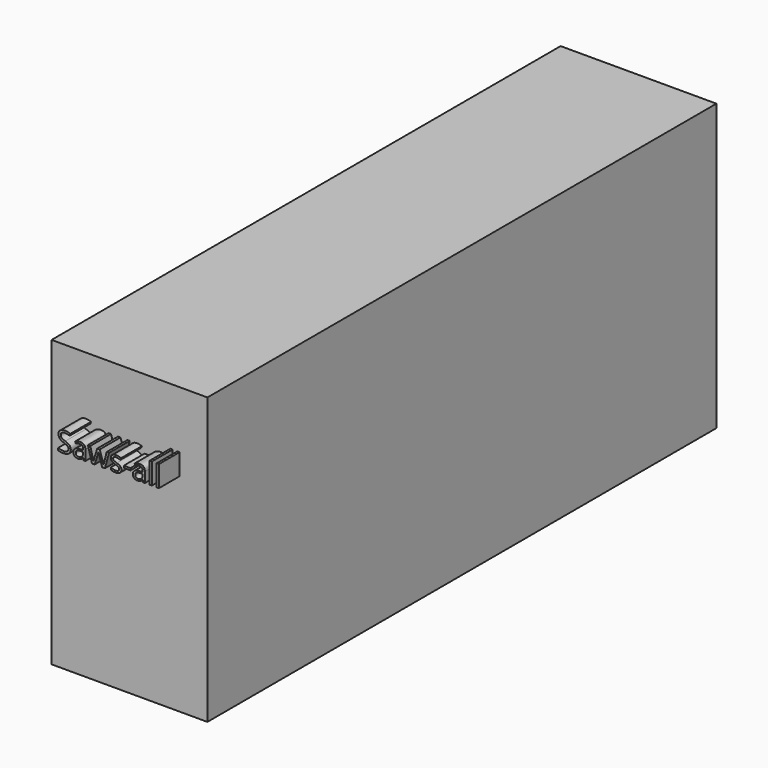
from build123d import *

# Parameters (mm, degrees)
F0_W         = 152.4
F0_H         = 279.4
F1_DEPTH     = 622.3
F2_TEXT_SIZE = 27.2934855608
F3_DEPTH     = 25.4


# Not quite as in the source:
# - Text() gives the source's letters only with a copy of the font that has no kerning and outlines rounded to 1/6400 em; it was checked with that copy


with BuildPart() as f1:
    # F0 (on Front) → F1 (new body)
    with BuildSketch(Plane.XZ):
        Rectangle(F0_W, F0_H)
    extrude(amount=F1_DEPTH)

    # F2 (on face) → F3 (join)
    with BuildSketch(Plane.XZ.offset(622.3)):
        with Locations((-50.8, 63.0063754654)):
            Text('Saws-all', F2_TEXT_SIZE, font='Open Sans', text_align=(TextAlign.LEFT, TextAlign.BOTTOM))
    extrude(amount=F3_DEPTH)


solid = f1.part
